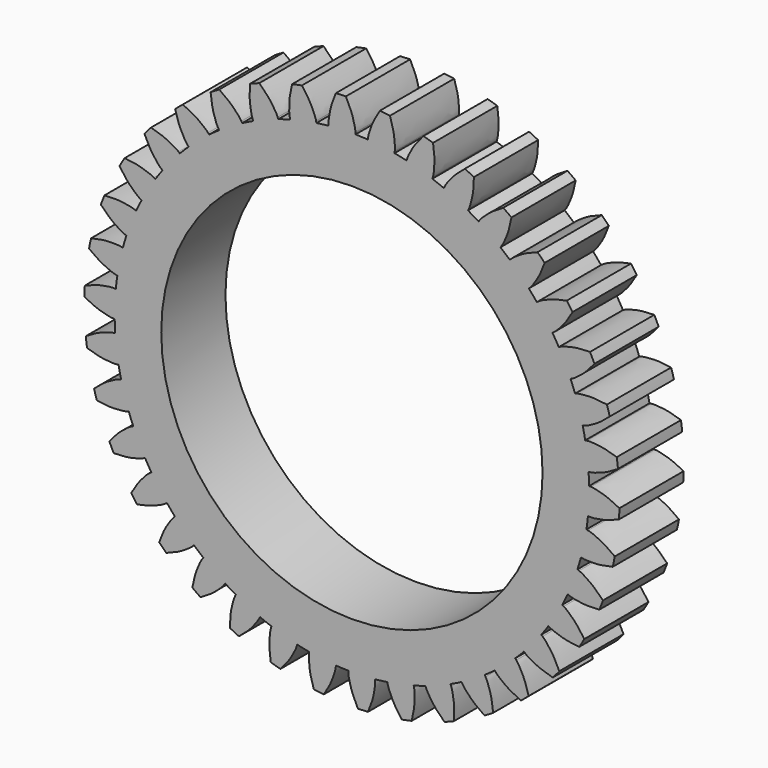
from build123d import *

# Parameters (mm, degrees)
F3_R            = 35.4587177464
F4_DEPTH        = 12
F6_DEPTH        = 12
F6_COPIES_COUNT = 38
F7_R            = 28.5
F8_DEPTH        = 12.0010001


# Not quite as in the source:
# - the dataset's text gives a spline's control points without its knots; the knots are read off the source's solid
# - a pattern or mirror of a feature is missing from the dataset's text; its kind, count and spacing are read off the source's solid


with BuildPart() as f4:
    # F3 (on Front) → F4 (new body)
    with BuildSketch(Plane.XZ):
        Circle(F3_R)
    extrude(amount=F4_DEPTH)

    # F5 (on Front) → F6 (join, through all)
    with BuildSketch(Plane.XZ):
        with BuildLine():
            ThreePointArc((-3.4687174361, 35.2886478002), (-1.4653305978, 35.4284274342), (0.5427565695, 35.4545635924))
            Line((0.5427565695, 35.4545635924), (0.5324253259, 35.704350032))
            add(Edge.make_bspline(
                [(-0.9026409231, 39.9898141952), (-0.6009721679, 39.4013724079), (0.0885099261, 38.0417669132), (0.5230456612, 36.1135725279), (0.5311372002, 35.7932176287), (0.5324253259, 35.704350032)],
                knots=[0.047563032, 0.047563032, 0.047563032, 0.047563032, 0.4365046984, 0.8342346014, 1, 1, 1, 1], degree=3))
            ThreePointArc((-0.9026409231, 39.9898141952), (-1.65299897, 39.9658303355), (-2.402774735, 39.9277682017))
            add(Edge.make_bspline(
                [(-2.402774735, 39.9277682017), (-2.6548200009, 39.3164246332), (-3.2296718321, 37.9045259005), (-3.5034943771, 35.9470336), (-3.4851035815, 35.6271046812), (-3.4790486797, 35.5384342398)],
                knots=[0.047563032, 0.047563032, 0.047563032, 0.047563032, 0.4365046984, 0.8342346014, 1, 1, 1, 1], degree=3))
            Line((-3.4790486797, 35.5384342398), (-3.4687174361, 35.2886478002))
        make_face()
    f6 = extrude(amount=F6_DEPTH)

    # F6_copies: F6 ×38 about axis
    f6_copies_axis = Axis((0, 0, 0), (0, 1, 0))
    for i in range(1, F6_COPIES_COUNT):
        add(f6.rotate(f6_copies_axis, i * 360 / F6_COPIES_COUNT))

    # F7 (on face) → F8 (cut, through all)
    with BuildSketch(Plane.XZ.offset(12)):
        Circle(F7_R)
    extrude(amount=-F8_DEPTH, mode=Mode.SUBTRACT)


solid = f4.part
